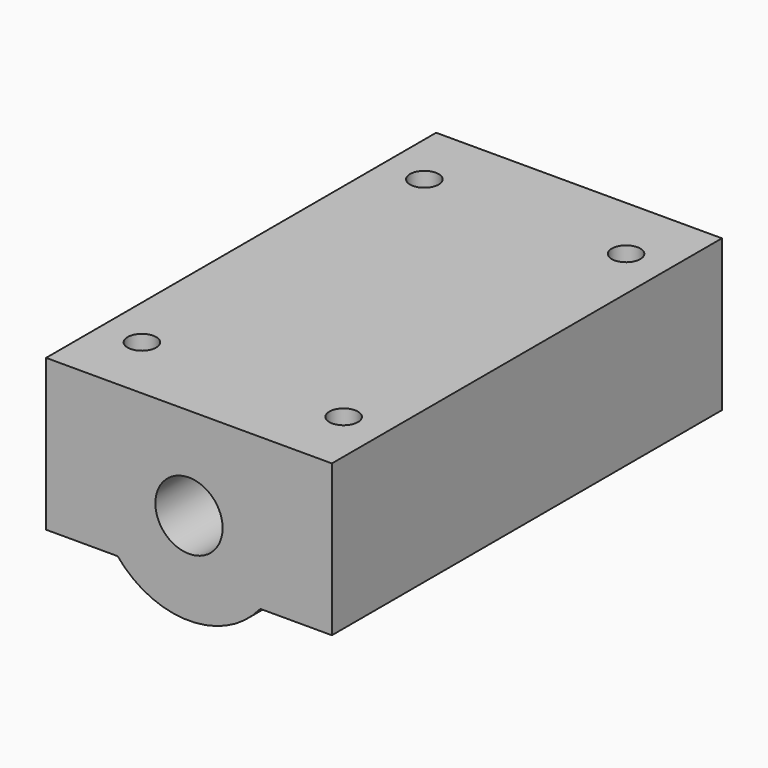
from build123d import *

# Parameters (mm, degrees)
F0_R     = 4
F1_DEPTH = 58
F2_R     = 1.7
F3_DEPTH = 11.001
F4_DEPTH = 11.001
F5_DEPTH = 50


# Not quite as in the source:
# - a feature names something its author has since deleted; it is built from what else it names


with BuildPart() as f1:
    # F0 (on Front) → F1 (new body)
    with BuildSketch(Plane.XZ):
        with BuildLine():
            Line((-17, -7), (-8.4852813742, -7))
            ThreePointArc((-8.4852813742, -7), (0, -11), (8.4852813742, -7))
            Line((8.4852813742, -7), (17, -7))
            Line((17, -7), (17, 11))
            Line((17, 11), (-17, 11))
            Line((-17, 11), (-17, -7))
        make_face()
        Circle(F0_R, mode=Mode.SUBTRACT)
    extrude(amount=F1_DEPTH)

    # F2 (on Top) → F3 (cut, through all)
    with BuildSketch(Plane.XY):
        with Locations((-12, -8)):
            Circle(F2_R)
        with Locations((12, -8)):
            Circle(F2_R)
        with Locations((12, -50)):
            Circle(F2_R)
        with Locations((-12, -50)):
            Circle(F2_R)
    extrude(amount=-F3_DEPTH, mode=Mode.SUBTRACT)

    # F2 (on Top) → F4 (cut, through all)
    with BuildSketch(Plane.XY):
        with Locations((-12, -8)):
            Circle(F2_R)
        with Locations((12, -8)):
            Circle(F2_R)
        with Locations((12, -50)):
            Circle(F2_R)
        with Locations((-12, -50)):
            Circle(F2_R)
    extrude(amount=-F4_DEPTH, mode=Mode.SUBTRACT)

    # F2 (on Top) → F5 (cut)
    with BuildSketch(Plane.XY):
        with Locations((-12, -8)):
            Circle(F2_R)
        with Locations((12, -8)):
            Circle(F2_R)
        with Locations((12, -50)):
            Circle(F2_R)
        with Locations((-12, -50)):
            Circle(F2_R)
    extrude(amount=F5_DEPTH, mode=Mode.SUBTRACT)


solid = f1.part
